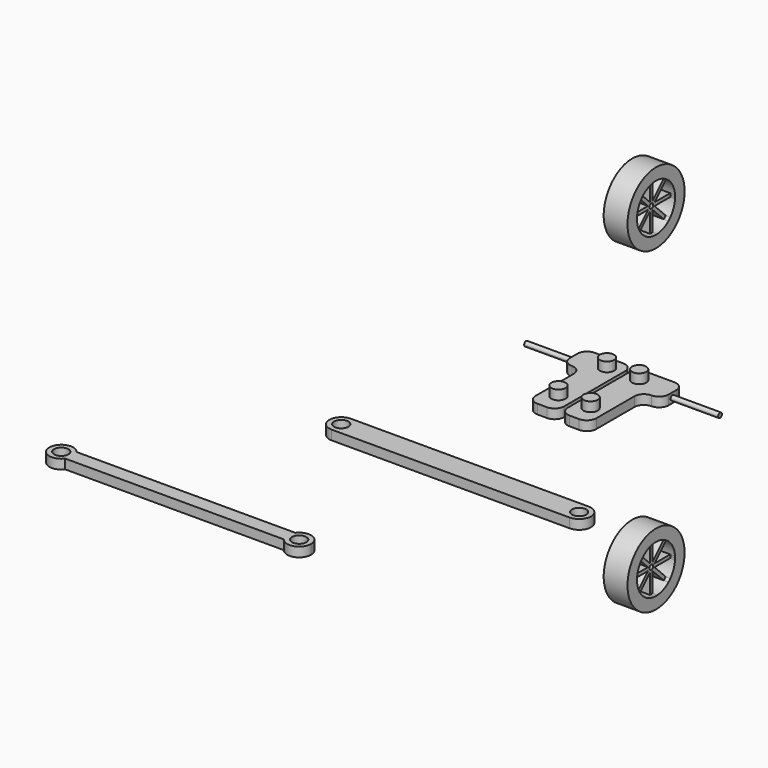
from build123d import *
from build123d import SkipClean  # not in build123d's __all__

# Parameters (mm, degrees)
F0_R      = 1.5
F1_DEPTH  = 2
F2_R      = 1.5
F3_DEPTH  = 2
F4_R      = 1.5
F5_DEPTH  = 4
F6_R      = 0.5
F7_DEPTH  = 10
F9_R      = 1.5
F10_DEPTH = 2
F11_R     = 7.5
F12_DEPTH = 5
F13_R     = 0.5
F14_DEPTH = 1
F15_R     = 0.5
F16_DEPTH = 1
F18_R     = 2
F19_R     = 1.99999
F20_R     = 1.99999


# Not quite as in the source:
# - a fillet or chamfer is up to 0.001 mm smaller than in the source, because OpenCascade refuses the exact size


with BuildPart() as f1:
    # F0 (on Top) → F1 (new body)
    with BuildSketch(Plane.XY):
        with BuildLine():
            Line((-25, 0), (0, 0))
            Line((0, 0), (25, 0))
            ThreePointArc((25, 0), (27.5, 2.5), (25, 5))
            Line((25, 5), (-25, 5))
            ThreePointArc((-25, 5), (-27.5, 2.5), (-25, 0))
        make_face()
        with Locations((-25, 2.5)):
            Circle(F0_R, mode=Mode.SUBTRACT)
        with Locations((25, 2.5)):
            Circle(F0_R, mode=Mode.SUBTRACT)
    extrude(amount=F1_DEPTH)


with BuildPart() as f3:
    # F2 (on Top) → F3 (new body)
    with BuildSketch(Plane.XY):
        Polygon((-0.3795566291, 28.2947075627), (-0.3795566291, 48.2947075627), (-10.3795566291, 48.2947075627), (-10.3795566291, 42.2947075627), (-6.3795566291, 42.2947075627), (-6.3795566291, 28.2947075627), align=None)
        with Locations((-3.3795566291, 32.5487554073)):
            Circle(F2_R, mode=Mode.SUBTRACT)
        with Locations((-3.3795566291, 45.2947075627)):
            Circle(F2_R, mode=Mode.SUBTRACT)
    extrude(amount=F3_DEPTH)

    # F4 (on Top) → F5 (join)
    with BuildSketch(Plane.XY):
        with Locations((-3.3795566291, 32.5487554073)):
            Circle(F4_R)
        with Locations((-3.3795566291, 45.2947075627)):
            Circle(F4_R)
    extrude(amount=F5_DEPTH)

    # F6 (on face) → F7 (join)
    with BuildSketch(Plane(origin=(-10.3795566291, 0, 0), x_dir=(0, -1, 0), z_dir=(-1, 0, 0))):
        with Locations((-45.2947075627, 1)):
            Circle(F6_R)
    extrude(amount=F7_DEPTH)


with BuildPart() as f8_1:
    # F8: instance of F3
    add(f3.part.mirror(Plane.YZ), clean=False)

    # F20 (radius 2 in the source; OpenCascade refuses exactly that, so slightly less here)
    f20_edges = [f8_1.edges().sort_by_distance(p)[0] for p in [
        (0.379557, 48.294708, 1),
        (10.379557, 48.294708, 1),
        (10.379557, 42.294708, 1),
        (6.379557, 28.294708, 1),
        (0.379557, 28.294708, 1),
        (6.379557, 42.294708, 1),
    ]]
    fillet(f20_edges, radius=F20_R)


with BuildPart() as f10:
    # F9 (on Top) → F10 (new body)
    with BuildSketch(Plane.XY):
        with BuildLine():
            ThreePointArc((-52.7561821239, -35.3634960353), (-52.3844738788, -34.6540654504), (-52.2561821239, -33.8634960353))
            ThreePointArc((-52.2561821239, -33.8634960353), (-52.3844738788, -33.0729266203), (-52.7561821239, -32.3634960353))
            ThreePointArc((-52.7561821239, -32.3634960353), (-57.2561821239, -33.8634960353), (-52.7561821239, -35.3634960353))
        make_face()
        with Locations((-54.7561821239, -33.8634960353)):
            Circle(F9_R, mode=Mode.SUBTRACT)
        with BuildLine():
            ThreePointArc((-52.7561821239, -32.3634960353), (-52.3844738788, -33.0729266203), (-52.2561821239, -33.8634960353))
            ThreePointArc((-52.2561821239, -33.8634960353), (-52.3844738788, -34.6540654504), (-52.7561821239, -35.3634960353))
            Line((-52.7561821239, -35.3634960353), (-6.7561821239, -35.3634960353))
            ThreePointArc((-6.7561821239, -35.3634960353), (-7.2561821239, -33.8634960353), (-6.7561821239, -32.3634960353))
            Line((-6.7561821239, -32.3634960353), (-52.7561821239, -32.3634960353))
        make_face()
        with BuildLine():
            ThreePointArc((-2.2561821239, -33.8634960353), (-3.9656127089, -31.4917877902), (-6.7561821239, -32.3634960353))
            ThreePointArc((-6.7561821239, -32.3634960353), (-7.2561821239, -33.8634960353), (-6.7561821239, -35.3634960353))
            ThreePointArc((-6.7561821239, -35.3634960353), (-3.9656127089, -36.2352042805), (-2.2561821239, -33.8634960353))
        make_face()
        with Locations((-4.7561821239, -33.8634960353)):
            Circle(F9_R, mode=Mode.SUBTRACT)
    extrude(amount=F10_DEPTH)


with BuildPart() as f12:
    # F11 (on Right) → F12 (new body)
    with BuildSketch(Plane.YZ):
        with Locations((47.7053249894, -33.4185645311)):
            Circle(F11_R)
        with BuildLine():
            ThreePointArc((52.6928093252, -33.0650111405), (52.7021950938, -33.2416771079), (52.7053249894, -33.4185645311))
            ThreePointArc((52.7053249894, -33.4185645311), (52.7021950938, -33.5954519542), (52.6928093252, -33.7721179217))
            ThreePointArc((52.6928093252, -33.7721179217), (52.324722652, -35.3319816929), (51.4820089843, -36.695248526))
            ThreePointArc((51.4820089843, -36.695248526), (51.3637240213, -36.8268069701), (51.2408588954, -36.954098437))
            ThreePointArc((51.2408588954, -36.954098437), (51.1135674285, -37.076963563), (50.9820089843, -37.195248526))
            ThreePointArc((50.9820089843, -37.195248526), (49.6187421513, -38.0379621936), (48.05887838, -38.4060488669))
            ThreePointArc((48.05887838, -38.4060488669), (47.8822124126, -38.4154346354), (47.7053249894, -38.4185645311))
            ThreePointArc((47.7053249894, -38.4185645311), (47.5284375663, -38.4154346354), (47.3517715988, -38.4060488669))
            ThreePointArc((47.3517715988, -38.4060488669), (45.7919078276, -38.0379621936), (44.4286409945, -37.195248526))
            ThreePointArc((44.4286409945, -37.195248526), (44.2970825504, -37.076963563), (44.1697910835, -36.954098437))
            ThreePointArc((44.1697910835, -36.954098437), (44.0469259575, -36.8268069701), (43.9286409945, -36.695248526))
            ThreePointArc((43.9286409945, -36.695248526), (43.0859273269, -35.3319816929), (42.7178406536, -33.7721179217))
            ThreePointArc((42.7178406536, -33.7721179217), (42.7084548851, -33.5954519542), (42.7053249894, -33.4185645311))
            ThreePointArc((42.7053249894, -33.4185645311), (42.7084548851, -33.2416771079), (42.7178406536, -33.0650111405))
            ThreePointArc((42.7178406536, -33.0650111405), (43.0859273269, -31.5051473692), (43.9286409945, -30.1418805362))
            ThreePointArc((43.9286409945, -30.1418805362), (44.0469259575, -30.010322092), (44.1697910835, -29.8830306251))
            ThreePointArc((44.1697910835, -29.8830306251), (44.2970825504, -29.7601654992), (44.4286409945, -29.6418805362))
            ThreePointArc((44.4286409945, -29.6418805362), (45.7919078276, -28.7991668685), (47.3517715988, -28.4310801953))
            ThreePointArc((47.3517715988, -28.4310801953), (47.5284375663, -28.4216944267), (47.7053249894, -28.4185645311))
            ThreePointArc((47.7053249894, -28.4185645311), (47.8822124126, -28.4216944267), (48.05887838, -28.4310801953))
            ThreePointArc((48.05887838, -28.4310801953), (49.6187421513, -28.7991668685), (50.9820089843, -29.6418805362))
            ThreePointArc((50.9820089843, -29.6418805362), (51.1135674285, -29.7601654992), (51.2408588954, -29.8830306251))
            ThreePointArc((51.2408588954, -29.8830306251), (51.3637240213, -30.010322092), (51.4820089843, -30.1418805362))
            ThreePointArc((51.4820089843, -30.1418805362), (52.324722652, -31.5051473692), (52.6928093252, -33.0650111405))
        make_face(mode=Mode.SUBTRACT)
        with BuildLine():
            Line((48.05887838, -32.5650111405), (48.05887838, -33.0650111405))
            Line((48.05887838, -33.0650111405), (51.2408588954, -29.8830306251))
            ThreePointArc((51.2408588954, -29.8830306251), (51.1135674285, -29.7601654992), (50.9820089843, -29.6418805362))
            Line((50.9820089843, -29.6418805362), (48.05887838, -32.5650111405))
        make_face()
        with BuildLine():
            Line((51.2408588954, -29.8830306251), (48.05887838, -33.0650111405))
            Line((48.05887838, -33.0650111405), (48.55887838, -33.0650111405))
            Line((48.55887838, -33.0650111405), (51.4820089843, -30.1418805362))
            ThreePointArc((51.4820089843, -30.1418805362), (51.3637240213, -30.010322092), (51.2408588954, -29.8830306251))
        make_face()
        with BuildLine():
            Line((47.7053249894, -28.4185645311), (47.7053249894, -32.9185645311))
            Line((47.7053249894, -32.9185645311), (48.05887838, -32.5650111405))
            Line((48.05887838, -32.5650111405), (48.05887838, -28.4310801953))
            ThreePointArc((48.05887838, -28.4310801953), (47.8822124126, -28.4216944267), (47.7053249894, -28.4185645311))
        make_face()
        with BuildLine():
            Line((47.3517715988, -32.5650111405), (47.7053249894, -32.9185645311))
            Line((47.7053249894, -32.9185645311), (47.7053249894, -28.4185645311))
            ThreePointArc((47.7053249894, -28.4185645311), (47.5284375663, -28.4216944267), (47.3517715988, -28.4310801953))
            Line((47.3517715988, -28.4310801953), (47.3517715988, -32.5650111405))
        make_face()
        with BuildLine():
            Line((44.1697910835, -29.8830306251), (47.3517715988, -33.0650111405))
            Line((47.3517715988, -33.0650111405), (47.3517715988, -32.5650111405))
            Line((47.3517715988, -32.5650111405), (44.4286409945, -29.6418805362))
            ThreePointArc((44.4286409945, -29.6418805362), (44.2970825504, -29.7601654992), (44.1697910835, -29.8830306251))
        make_face()
        with BuildLine():
            Line((46.8517715988, -33.0650111405), (47.3517715988, -33.0650111405))
            Line((47.3517715988, -33.0650111405), (44.1697910835, -29.8830306251))
            ThreePointArc((44.1697910835, -29.8830306251), (44.0469259575, -30.010322092), (43.9286409945, -30.1418805362))
            Line((43.9286409945, -30.1418805362), (46.8517715988, -33.0650111405))
        make_face()
        with BuildLine():
            Line((42.7053249894, -33.4185645311), (47.2053249894, -33.4185645311))
            Line((47.2053249894, -33.4185645311), (46.8517715988, -33.0650111405))
            Line((46.8517715988, -33.0650111405), (42.7178406536, -33.0650111405))
            ThreePointArc((42.7178406536, -33.0650111405), (42.7084548851, -33.2416771079), (42.7053249894, -33.4185645311))
        make_face()
        with BuildLine():
            Line((46.8517715988, -33.7721179217), (47.2053249894, -33.4185645311))
            Line((47.2053249894, -33.4185645311), (42.7053249894, -33.4185645311))
            ThreePointArc((42.7053249894, -33.4185645311), (42.7084548851, -33.5954519542), (42.7178406536, -33.7721179217))
            Line((42.7178406536, -33.7721179217), (46.8517715988, -33.7721179217))
        make_face()
        with BuildLine():
            ThreePointArc((47.3517715988, -33.0650111405), (47.5139832732, -32.9566247648), (47.7053249894, -32.9185645311))
            Line((47.7053249894, -32.9185645311), (47.3517715988, -32.5650111405))
            Line((47.3517715988, -32.5650111405), (47.3517715988, -33.0650111405))
        make_face()
        with BuildLine():
            ThreePointArc((47.7053249894, -32.9185645311), (47.8966667056, -32.9566247648), (48.05887838, -33.0650111405))
            Line((48.05887838, -33.0650111405), (48.05887838, -32.5650111405))
            Line((48.05887838, -32.5650111405), (47.7053249894, -32.9185645311))
        make_face()
        with BuildLine():
            ThreePointArc((48.05887838, -33.0650111405), (48.1672647557, -33.2272228149), (48.2053249894, -33.4185645311))
            Line((48.2053249894, -33.4185645311), (48.55887838, -33.0650111405))
            Line((48.55887838, -33.0650111405), (48.05887838, -33.0650111405))
        make_face()
        with BuildLine():
            Line((48.55887838, -33.7721179217), (48.2053249894, -33.4185645311))
            ThreePointArc((48.2053249894, -33.4185645311), (48.1672647557, -33.6099062473), (48.05887838, -33.7721179217))
            Line((48.05887838, -33.7721179217), (48.55887838, -33.7721179217))
        make_face()
        with BuildLine():
            Line((48.05887838, -34.2721179217), (48.05887838, -33.7721179217))
            ThreePointArc((48.05887838, -33.7721179217), (47.8966667056, -33.8805042973), (47.7053249894, -33.9185645311))
            Line((47.7053249894, -33.9185645311), (48.05887838, -34.2721179217))
        make_face()
        with BuildLine():
            Line((47.3517715988, -34.2721179217), (47.7053249894, -33.9185645311))
            ThreePointArc((47.7053249894, -33.9185645311), (47.5139832732, -33.8805042973), (47.3517715988, -33.7721179217))
            Line((47.3517715988, -33.7721179217), (47.3517715988, -34.2721179217))
        make_face()
        with BuildLine():
            ThreePointArc((47.3517715988, -33.7721179217), (47.2433852232, -33.6099062473), (47.2053249894, -33.4185645311))
            Line((47.2053249894, -33.4185645311), (46.8517715988, -33.7721179217))
            Line((46.8517715988, -33.7721179217), (47.3517715988, -33.7721179217))
        make_face()
        with BuildLine():
            Line((46.8517715988, -33.0650111405), (47.2053249894, -33.4185645311))
            ThreePointArc((47.2053249894, -33.4185645311), (47.2433852232, -33.2272228149), (47.3517715988, -33.0650111405))
            Line((47.3517715988, -33.0650111405), (46.8517715988, -33.0650111405))
        make_face()
        with BuildLine():
            Line((44.1697910835, -36.954098437), (47.3517715988, -33.7721179217))
            Line((47.3517715988, -33.7721179217), (46.8517715988, -33.7721179217))
            Line((46.8517715988, -33.7721179217), (43.9286409945, -36.695248526))
            ThreePointArc((43.9286409945, -36.695248526), (44.0469259575, -36.8268069701), (44.1697910835, -36.954098437))
        make_face()
        with BuildLine():
            Line((47.3517715988, -34.2721179217), (47.3517715988, -33.7721179217))
            Line((47.3517715988, -33.7721179217), (44.1697910835, -36.954098437))
            ThreePointArc((44.1697910835, -36.954098437), (44.2970825504, -37.076963563), (44.4286409945, -37.195248526))
            Line((44.4286409945, -37.195248526), (47.3517715988, -34.2721179217))
        make_face()
        with BuildLine():
            Line((47.7053249894, -38.4185645311), (47.7053249894, -33.9185645311))
            Line((47.7053249894, -33.9185645311), (47.3517715988, -34.2721179217))
            Line((47.3517715988, -34.2721179217), (47.3517715988, -38.4060488669))
            ThreePointArc((47.3517715988, -38.4060488669), (47.5284375663, -38.4154346354), (47.7053249894, -38.4185645311))
        make_face()
        with BuildLine():
            Line((48.05887838, -34.2721179217), (47.7053249894, -33.9185645311))
            Line((47.7053249894, -33.9185645311), (47.7053249894, -38.4185645311))
            ThreePointArc((47.7053249894, -38.4185645311), (47.8822124126, -38.4154346354), (48.05887838, -38.4060488669))
            Line((48.05887838, -38.4060488669), (48.05887838, -34.2721179217))
        make_face()
        with BuildLine():
            Line((51.2408588954, -36.954098437), (48.05887838, -33.7721179217))
            Line((48.05887838, -33.7721179217), (48.05887838, -34.2721179217))
            Line((48.05887838, -34.2721179217), (50.9820089843, -37.195248526))
            ThreePointArc((50.9820089843, -37.195248526), (51.1135674285, -37.076963563), (51.2408588954, -36.954098437))
        make_face()
        with BuildLine():
            Line((48.55887838, -33.7721179217), (48.05887838, -33.7721179217))
            Line((48.05887838, -33.7721179217), (51.2408588954, -36.954098437))
            ThreePointArc((51.2408588954, -36.954098437), (51.3637240213, -36.8268069701), (51.4820089843, -36.695248526))
            Line((51.4820089843, -36.695248526), (48.55887838, -33.7721179217))
        make_face()
        with BuildLine():
            Line((52.7053249894, -33.4185645311), (48.2053249894, -33.4185645311))
            Line((48.2053249894, -33.4185645311), (48.55887838, -33.7721179217))
            Line((48.55887838, -33.7721179217), (52.6928093252, -33.7721179217))
            ThreePointArc((52.6928093252, -33.7721179217), (52.7021950938, -33.5954519542), (52.7053249894, -33.4185645311))
        make_face()
        with BuildLine():
            Line((48.55887838, -33.0650111405), (48.2053249894, -33.4185645311))
            Line((48.2053249894, -33.4185645311), (52.7053249894, -33.4185645311))
            ThreePointArc((52.7053249894, -33.4185645311), (52.7021950938, -33.2416771079), (52.6928093252, -33.0650111405))
            Line((52.6928093252, -33.0650111405), (48.55887838, -33.0650111405))
        make_face()
    extrude(amount=F12_DEPTH)

    # F13 (on face) → F14 (cut)
    with BuildSketch(Plane(origin=(0, 0, 0), x_dir=(0, -1, 0), z_dir=(-1, 0, 0))):
        with BuildLine():
            ThreePointArc((-48.05887838, -28.4310801953), (-49.6187421513, -28.7991668685), (-50.9820089843, -29.6418805362))
            Line((-50.9820089843, -29.6418805362), (-48.05887838, -32.5650111405))
            Line((-48.05887838, -32.5650111405), (-48.05887838, -28.4310801953))
        make_face()
        with BuildLine():
            Line((-48.05887838, -32.5650111405), (-50.9820089843, -29.6418805362))
            ThreePointArc((-50.9820089843, -29.6418805362), (-51.2408588954, -29.8830306251), (-51.4820089843, -30.1418805362))
            Line((-51.4820089843, -30.1418805362), (-48.55887838, -33.0650111405))
            Line((-48.55887838, -33.0650111405), (-52.6928093252, -33.0650111405))
            ThreePointArc((-52.6928093252, -33.0650111405), (-52.7053249894, -33.4185645311), (-52.6928093252, -33.7721179217))
            Line((-52.6928093252, -33.7721179217), (-48.55887838, -33.7721179217))
            Line((-48.55887838, -33.7721179217), (-51.4820089843, -36.695248526))
            ThreePointArc((-51.4820089843, -36.695248526), (-51.2408588954, -36.954098437), (-50.9820089843, -37.195248526))
            ThreePointArc((-50.9820089843, -37.195248526), (-49.6187421513, -38.0379621936), (-48.05887838, -38.4060488669))
            ThreePointArc((-48.05887838, -38.4060488669), (-47.7053249894, -38.4185645311), (-47.3517715988, -38.4060488669))
            Line((-47.3517715988, -38.4060488669), (-47.3517715988, -34.2721179217))
            Line((-47.3517715988, -34.2721179217), (-44.4286409945, -37.195248526))
            ThreePointArc((-44.4286409945, -37.195248526), (-44.1697910835, -36.954098437), (-43.9286409945, -36.695248526))
            Line((-43.9286409945, -36.695248526), (-46.8517715988, -33.7721179217))
            Line((-46.8517715988, -33.7721179217), (-42.7178406536, -33.7721179217))
            ThreePointArc((-42.7178406536, -33.7721179217), (-42.7084548851, -33.5954519542), (-42.7053249894, -33.4185645311))
            ThreePointArc((-42.7053249894, -33.4185645311), (-42.7084548851, -33.2416771079), (-42.7178406536, -33.0650111405))
            Line((-42.7178406536, -33.0650111405), (-46.8517715988, -33.0650111405))
            Line((-46.8517715988, -33.0650111405), (-43.9286409945, -30.1418805362))
            ThreePointArc((-43.9286409945, -30.1418805362), (-44.1697910835, -29.8830306251), (-44.4286409945, -29.6418805362))
            Line((-44.4286409945, -29.6418805362), (-47.3517715988, -32.5650111405))
            Line((-47.3517715988, -32.5650111405), (-47.3517715988, -28.4310801953))
            ThreePointArc((-47.3517715988, -28.4310801953), (-47.7053249894, -28.4185645311), (-48.05887838, -28.4310801953))
            Line((-48.05887838, -28.4310801953), (-48.05887838, -32.5650111405))
        make_face()
        with Locations((-47.7053249894, -33.4185645311)):
            Circle(F13_R, mode=Mode.SUBTRACT)
        with BuildLine():
            Line((-48.55887838, -33.0650111405), (-51.4820089843, -30.1418805362))
            ThreePointArc((-51.4820089843, -30.1418805362), (-52.324722652, -31.5051473692), (-52.6928093252, -33.0650111405))
            Line((-52.6928093252, -33.0650111405), (-48.55887838, -33.0650111405))
        make_face()
        with BuildLine():
            ThreePointArc((-44.4286409945, -29.6418805362), (-45.7919078276, -28.7991668685), (-47.3517715988, -28.4310801953))
            Line((-47.3517715988, -28.4310801953), (-47.3517715988, -32.5650111405))
            Line((-47.3517715988, -32.5650111405), (-44.4286409945, -29.6418805362))
        make_face()
        with BuildLine():
            Line((-48.55887838, -33.7721179217), (-52.6928093252, -33.7721179217))
            ThreePointArc((-52.6928093252, -33.7721179217), (-52.324722652, -35.3319816929), (-51.4820089843, -36.695248526))
            Line((-51.4820089843, -36.695248526), (-48.55887838, -33.7721179217))
        make_face()
        with BuildLine():
            ThreePointArc((-42.7178406536, -33.0650111405), (-43.0859273269, -31.5051473692), (-43.9286409945, -30.1418805362))
            Line((-43.9286409945, -30.1418805362), (-46.8517715988, -33.0650111405))
            Line((-46.8517715988, -33.0650111405), (-42.7178406536, -33.0650111405))
        make_face()
        with BuildLine():
            ThreePointArc((-43.9286409945, -36.695248526), (-43.0859273269, -35.3319816929), (-42.7178406536, -33.7721179217))
            Line((-42.7178406536, -33.7721179217), (-46.8517715988, -33.7721179217))
            Line((-46.8517715988, -33.7721179217), (-43.9286409945, -36.695248526))
        make_face()
        with BuildLine():
            Line((-47.3517715988, -34.2721179217), (-47.3517715988, -38.4060488669))
            ThreePointArc((-47.3517715988, -38.4060488669), (-45.7919078276, -38.0379621936), (-44.4286409945, -37.195248526))
            Line((-44.4286409945, -37.195248526), (-47.3517715988, -34.2721179217))
        make_face()
        with Locations((-47.7053249894, -33.4185645311)):
            Circle(F13_R)
    with SkipClean():  # cleaning this boolean's faces spoils the solid; the shape is the same uncleaned
        extrude(amount=-F14_DEPTH, mode=Mode.SUBTRACT)

    # F15 (on face) → F16 (cut)
    with BuildSketch(Plane.YZ.offset(5)):
        with BuildLine():
            ThreePointArc((51.4820089843, -30.1418805362), (51.2408588954, -29.8830306251), (50.9820089843, -29.6418805362))
            Line((50.9820089843, -29.6418805362), (48.05887838, -32.5650111405))
            Line((48.05887838, -32.5650111405), (48.05887838, -28.4310801953))
            ThreePointArc((48.05887838, -28.4310801953), (47.7053249894, -28.4185645311), (47.3517715988, -28.4310801953))
            Line((47.3517715988, -28.4310801953), (47.3517715988, -32.5650111405))
            Line((47.3517715988, -32.5650111405), (44.4286409945, -29.6418805362))
            ThreePointArc((44.4286409945, -29.6418805362), (44.1697910835, -29.8830306251), (43.9286409945, -30.1418805362))
            Line((43.9286409945, -30.1418805362), (46.8517715988, -33.0650111405))
            Line((46.8517715988, -33.0650111405), (42.7178406536, -33.0650111405))
            ThreePointArc((42.7178406536, -33.0650111405), (42.7053249894, -33.4185645311), (42.7178406536, -33.7721179217))
            Line((42.7178406536, -33.7721179217), (46.8517715988, -33.7721179217))
            Line((46.8517715988, -33.7721179217), (43.9286409945, -36.695248526))
            ThreePointArc((43.9286409945, -36.695248526), (44.1697910835, -36.954098437), (44.4286409945, -37.195248526))
            Line((44.4286409945, -37.195248526), (47.3517715988, -34.2721179217))
            Line((47.3517715988, -34.2721179217), (47.3517715988, -38.4060488669))
            ThreePointArc((47.3517715988, -38.4060488669), (47.7053249894, -38.4185645311), (48.05887838, -38.4060488669))
            Line((48.05887838, -38.4060488669), (48.05887838, -34.2721179217))
            Line((48.05887838, -34.2721179217), (50.9820089843, -37.195248526))
            ThreePointArc((50.9820089843, -37.195248526), (51.2408588954, -36.954098437), (51.4820089843, -36.695248526))
            Line((51.4820089843, -36.695248526), (48.55887838, -33.7721179217))
            Line((48.55887838, -33.7721179217), (52.6928093252, -33.7721179217))
            ThreePointArc((52.6928093252, -33.7721179217), (52.7021950938, -33.5954519542), (52.7053249894, -33.4185645311))
            ThreePointArc((52.7053249894, -33.4185645311), (52.7021950938, -33.2416771079), (52.6928093252, -33.0650111405))
            Line((52.6928093252, -33.0650111405), (48.55887838, -33.0650111405))
            Line((48.55887838, -33.0650111405), (51.4820089843, -30.1418805362))
        make_face()
        with Locations((47.7053249894, -33.4185645311)):
            Circle(F15_R, mode=Mode.SUBTRACT)
    with SkipClean():  # cleaning this boolean's faces spoils the solid; the shape is the same uncleaned
        extrude(amount=-F16_DEPTH, mode=Mode.SUBTRACT)


with BuildPart() as f17_1:
    # F17: instance of F12
    add(f12.part.mirror(Plane.XY), clean=False)


with BuildPart() as f3_1:
    add(f3.part, clean=False)

    # F18
    f18_edges = [f3_1.edges().sort_by_distance(p)[0] for p in [
        (-10.379557, 48.294708, 1),
    ]]
    fillet(f18_edges, radius=F18_R)

    # F19 (radius 2 in the source; OpenCascade refuses exactly that, so slightly less here)
    f19_edges = [f3_1.edges().sort_by_distance(p)[0] for p in [
        (-10.379557, 42.294708, 1),
        (-6.379557, 42.294708, 1),
        (-6.379557, 28.294708, 1),
        (-0.379557, 28.294708, 1),
        (-0.379557, 48.294708, 1),
    ]]
    fillet(f19_edges, radius=F19_R)


solid = Compound([f1.part, f8_1.part, f10.part, f12.part, f17_1.part, f3_1.part])
